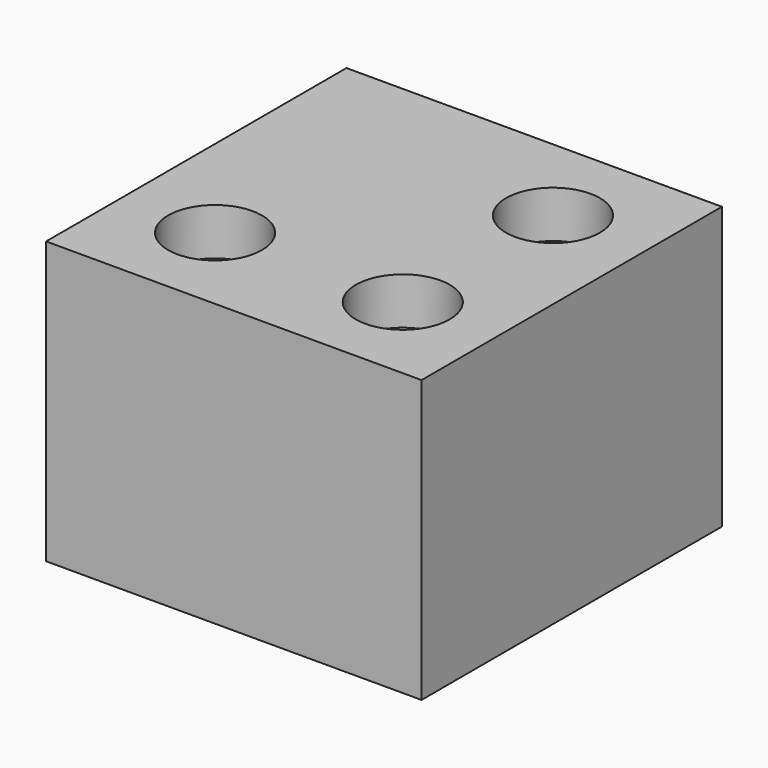
from build123d import *

# Parameters (mm, degrees)
F0_W     = 32
F0_H     = 32
F1_DEPTH = 20
F4_W     = 32
F4_H     = 32
F4_R     = 4
F5_DEPTH = 4


# Not quite as in the source:
# - the program builds the solid bodies; features that only make, move or delete a surface that nothing else refers to are left out


with BuildPart() as f1:
    # F0 (on Top) → F1 (new body)
    with BuildSketch(Plane.XY):
        with Locations((21.8166250885, -5.5067900717)):
            Rectangle(F0_W, F0_H)
    extrude(amount=F1_DEPTH)

    # F4 (on face) → F5 (join)
    with BuildSketch(Plane.XY.offset(20)):
        with Locations((21.8166250885, -5.5067900717)):
            Rectangle(F4_W, F4_H)
        with Locations((13.8166250885, -13.5067900717)):
            Circle(F4_R, mode=Mode.SUBTRACT)
        with Locations((29.8166250885, -13.5067900717)):
            Circle(F4_R, mode=Mode.SUBTRACT)
        with Locations((29.8166250885, 2.4932099283)):
            Circle(F4_R, mode=Mode.SUBTRACT)
    extrude(amount=F5_DEPTH)


solid = f1.part
